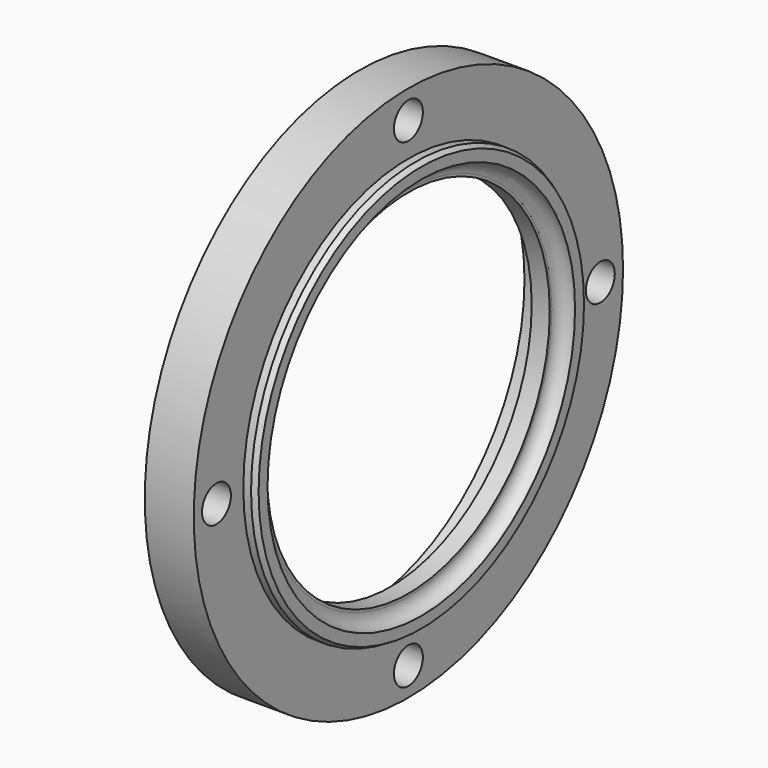
from build123d import *

# Parameters (mm, degrees)
F0_R     = 104
F0_R_2   = 68.5
F1_DEPTH = 19
F2_R     = 80
F2_R_2   = 74.5
F3_DEPTH = 5
F4_R     = 80
F5_DEPTH = 12
F6_SIZE2 = 1.1547005384
F6_SIZE  = 2
F7_R     = 4.99999
F9_D     = 14
F9_DEPTH = 25.5
F9_TIP   = 4.2060243332


# Not quite as in the source:
# - a fillet or chamfer is up to 0.001 mm smaller than in the source, because OpenCascade refuses the exact size


with BuildPart() as f1:
    # F0 (on Right) → F1 (new body)
    with BuildSketch(Plane.YZ):
        Circle(F0_R)
        Circle(F0_R_2, mode=Mode.SUBTRACT)
    extrude(amount=-F1_DEPTH)

    # F2 (on face) → F3 (join)
    with BuildSketch(Plane.YZ):
        Circle(F2_R)
        Circle(F2_R_2, mode=Mode.SUBTRACT)
    extrude(amount=F3_DEPTH)

    # F4 (on face) → F5 (cut)
    with BuildSketch(Plane(origin=(-19, 0, 0), x_dir=(0, -1, 0), z_dir=(-1, 0, 0))):
        Circle(F4_R)
    extrude(amount=-F5_DEPTH, mode=Mode.SUBTRACT)

    # F6
    f6_edges = [f1.edges().sort_by_distance(p)[0] for p in [
        (5, -80, 0),
    ]]
    f6_side = f1.faces().sort_by_distance((2.5, -80, 0))[0]
    chamfer(f6_edges, length=F6_SIZE, length2=F6_SIZE2, reference=f6_side)

    # F7 (radius 5 in the source; OpenCascade refuses exactly that, so slightly less here)
    f7_edges = [f1.edges().sort_by_distance(p)[0] for p in [
        (0, -74.5, 0),
    ]]
    fillet(f7_edges, radius=F7_R)

    # F9
    with Locations(Plane(origin=(-19, 0, 0), x_dir=(0, -1, 0), z_dir=(-1, 0, 0))):
        with Locations((0, -93), (-93, 0), (0, 93), (93, 0)):
            Hole(F9_D / 2, depth=F9_DEPTH)
            with Locations((0, 0, -(F9_DEPTH + F9_TIP / 2))):  # 118° drill point
                Cone(0, F9_D / 2, F9_TIP, mode=Mode.SUBTRACT)


solid = f1.part
